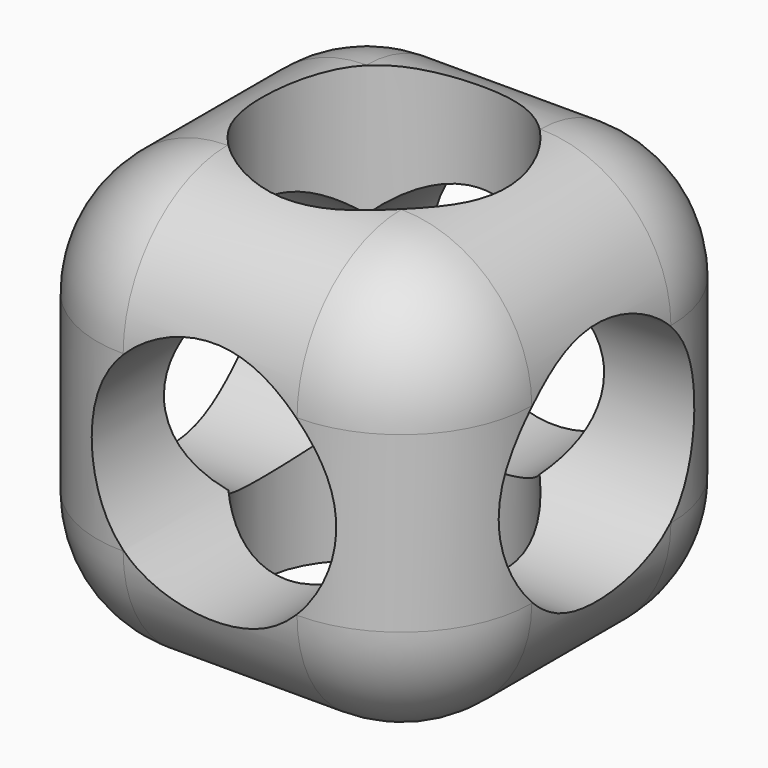
from build123d import *

# Parameters (mm, degrees)
F0_W         = 25.4
F0_H         = 25.4
F1_DEPTH     = 12.7
F5_D         = 14.2875
F5_ON_F3_D   = 14.2875
F5_ON_F2_D   = 14.2875
F6_T1_DEPTH  = 10.16
F6_T3_DEPTH  = 10.16
F6_T5_DEPTH  = 10.16
F6_S9_W      = 7.62
F6_S9_H      = 7.62
F6_T10_DEPTH = 7.62
F6_S15_W     = 7.62
F6_S15_H     = 7.62
F6_T16_DEPTH = 7.62
F6_S21_W     = 7.62
F6_S21_H     = 7.62
F6_T22_DEPTH = 7.62
F6_S27_W     = 7.62
F6_S27_H     = 7.62
F6_T28_DEPTH = 7.62
F6_S33_W     = 7.62
F6_S33_H     = 7.62
F6_T34_DEPTH = 7.62
F6_S39_W     = 7.62
F6_S39_H     = 7.62
F6_T40_DEPTH = 7.62
F6_S45_W     = 7.62
F6_S45_H     = 7.62
F6_T46_DEPTH = 7.62
F6_S51_W     = 7.62
F6_S51_H     = 7.62
F6_T52_DEPTH = 7.62


# Not quite as in the source:
# - a fillet or chamfer that OpenCascade refuses, or shapes differently, is made with other operations: its cross-section is extruded or revolved along the edge and cut away or added
# - a length typed as a fraction of an inch, garbled in the dataset ("3 / 203.2 mm" for 3/8 in), is restored


with BuildPart() as f1:
    # F0 (on Front) → F1 (new body, symmetric)
    with BuildSketch(Plane.XZ):
        Rectangle(F0_W, F0_H)
    extrude(amount=F1_DEPTH, both=True)

    # F5 (through all)
    with Locations(Plane.XY.offset(12.7)):
        with Locations((0, 0)):
            Hole(F5_D / 2)

    # F5 on F3 (through all)
    with Locations(Plane.XZ.offset(12.7)):
        with Locations((0, 0)):
            Hole(F5_ON_F3_D / 2)

    # F5 on F2 (through all)
    with Locations(Plane.YZ.offset(12.7)):
        with Locations((0, 0)):
            Hole(F5_ON_F2_D / 2)

    # F6: fillet of radius 7.62 on 12 edges, made by hand

    # F6_s2 → F6_t1 (cut)
    with BuildSketch(Plane.XZ.offset(-5.08)):
        with BuildLine():
            ThreePointArc((12.7, 5.08), (10.4681536726, 10.4681536726), (5.08, 12.7))
            Line((5.08, 12.7), (12.7, 12.7))
            Line((12.7, 12.7), (12.7, 5.08))
        make_face()
        with BuildLine():
            ThreePointArc((12.7, -5.08), (10.4681536726, -10.4681536726), (5.08, -12.7))
            Line((5.08, -12.7), (12.7, -12.7))
            Line((12.7, -12.7), (12.7, -5.08))
        make_face()
        with BuildLine():
            ThreePointArc((-5.08, 12.7), (-10.4681536726, 10.4681536726), (-12.7, 5.08))
            Line((-12.7, 5.08), (-12.7, 12.7))
            Line((-12.7, 12.7), (-5.08, 12.7))
        make_face()
        with BuildLine():
            ThreePointArc((-5.08, -12.7), (-10.4681536726, -10.4681536726), (-12.7, -5.08))
            Line((-12.7, -5.08), (-12.7, -12.7))
            Line((-12.7, -12.7), (-5.08, -12.7))
        make_face()
    extrude(amount=F6_T1_DEPTH, mode=Mode.SUBTRACT)

    # F6_s4 → F6_t3 (cut)
    with BuildSketch(Plane.XY.offset(-5.08)):
        with BuildLine():
            ThreePointArc((12.7, 5.08), (10.4681536726, 10.4681536726), (5.08, 12.7))
            Line((5.08, 12.7), (12.7, 12.7))
            Line((12.7, 12.7), (12.7, 5.08))
        make_face()
        with BuildLine():
            ThreePointArc((12.7, -5.08), (10.4681536726, -10.4681536726), (5.08, -12.7))
            Line((5.08, -12.7), (12.7, -12.7))
            Line((12.7, -12.7), (12.7, -5.08))
        make_face()
        with BuildLine():
            ThreePointArc((-5.08, -12.7), (-10.4681536726, -10.4681536726), (-12.7, -5.08))
            Line((-12.7, -5.08), (-12.7, -12.7))
            Line((-12.7, -12.7), (-5.08, -12.7))
        make_face()
        with BuildLine():
            ThreePointArc((-5.08, 12.7), (-10.4681536726, 10.4681536726), (-12.7, 5.08))
            Line((-12.7, 5.08), (-12.7, 12.7))
            Line((-12.7, 12.7), (-5.08, 12.7))
        make_face()
    extrude(amount=F6_T3_DEPTH, mode=Mode.SUBTRACT)

    # F6_s6 → F6_t5 (cut)
    with BuildSketch(Plane.YZ.offset(-5.08)):
        with BuildLine():
            ThreePointArc((-5.08, 12.7), (-10.4681536726, 10.4681536726), (-12.7, 5.08))
            Line((-12.7, 5.08), (-12.7, 12.7))
            Line((-12.7, 12.7), (-5.08, 12.7))
        make_face()
        with BuildLine():
            ThreePointArc((-5.08, -12.7), (-10.4681536726, -10.4681536726), (-12.7, -5.08))
            Line((-12.7, -5.08), (-12.7, -12.7))
            Line((-12.7, -12.7), (-5.08, -12.7))
        make_face()
        with BuildLine():
            ThreePointArc((12.7, 5.08), (10.4681536726, 10.4681536726), (5.08, 12.7))
            Line((5.08, 12.7), (12.7, 12.7))
            Line((12.7, 12.7), (12.7, 5.08))
        make_face()
        with BuildLine():
            ThreePointArc((12.7, -5.08), (10.4681536726, -10.4681536726), (5.08, -12.7))
            Line((5.08, -12.7), (12.7, -12.7))
            Line((12.7, -12.7), (12.7, -5.08))
        make_face()
    extrude(amount=F6_T5_DEPTH, mode=Mode.SUBTRACT)


with BuildPart() as f6_tool8:
    # F6_s9 → F6_t10 (new body)
    with BuildSketch(Plane.YZ.offset(5.08)):
        with Locations((8.89, 8.89)):
            Rectangle(F6_S9_W, F6_S9_H)
    extrude(amount=F6_T10_DEPTH)

    # F6_s11 → F6_t12 (revolve, cut)
    with BuildSketch(Plane(origin=(5.08, 5.08, 5.08), x_dir=(0, -0.7071067812, -0.7071067812), z_dir=(0, -0.7071067812, 0.7071067812))):
        with BuildLine():
            ThreePointArc((0, -7.62), (7.62, 0), (0, 7.62))
            Line((0, 7.62), (0, -7.62))
        make_face()
    revolve(axis=Axis((5.08, 5.08, 5.08), (1, 0, 0)), mode=Mode.SUBTRACT)


with BuildPart() as f1_1:
    add(f1.part)

    # F6_t7: cut F6_tool8
    add(f6_tool8.part, mode=Mode.SUBTRACT)


with BuildPart() as f6_tool14:
    # F6_s15 → F6_t16 (new body)
    with BuildSketch(Plane.YZ.offset(5.08)):
        with Locations((-8.89, 8.89)):
            Rectangle(F6_S15_W, F6_S15_H)
    extrude(amount=F6_T16_DEPTH)

    # F6_s17 → F6_t18 (revolve, cut)
    with BuildSketch(Plane(origin=(5.08, -5.08, 5.08), x_dir=(0, 0.7071067812, -0.7071067812), z_dir=(0, -0.7071067812, -0.7071067812))):
        with BuildLine():
            ThreePointArc((0, -7.62), (7.62, 0), (0, 7.62))
            Line((0, 7.62), (0, -7.62))
        make_face()
    revolve(axis=Axis((5.08, -5.08, 5.08), (1, 0, 0)), mode=Mode.SUBTRACT)


with BuildPart() as f1_2:
    add(f1_1.part)

    # F6_t13: cut F6_tool14
    add(f6_tool14.part, mode=Mode.SUBTRACT)


with BuildPart() as f6_tool20:
    # F6_s21 → F6_t22 (new body)
    with BuildSketch(Plane.YZ.offset(5.08)):
        with Locations((-8.89, -8.89)):
            Rectangle(F6_S21_W, F6_S21_H)
    extrude(amount=F6_T22_DEPTH)

    # F6_s23 → F6_t24 (revolve, cut)
    with BuildSketch(Plane(origin=(5.08, -5.08, -5.08), x_dir=(0, 0.7071067812, 0.7071067812), z_dir=(0, 0.7071067812, -0.7071067812))):
        with BuildLine():
            ThreePointArc((0, -7.62), (7.62, 0), (0, 7.62))
            Line((0, 7.62), (0, -7.62))
        make_face()
    revolve(axis=Axis((5.08, -5.08, -5.08), (1, 0, 0)), mode=Mode.SUBTRACT)


with BuildPart() as f1_3:
    add(f1_2.part)

    # F6_t19: cut F6_tool20
    add(f6_tool20.part, mode=Mode.SUBTRACT)


with BuildPart() as f6_tool26:
    # F6_s27 → F6_t28 (new body)
    with BuildSketch(Plane.YZ.offset(5.08)):
        with Locations((8.89, -8.89)):
            Rectangle(F6_S27_W, F6_S27_H)
    extrude(amount=F6_T28_DEPTH)

    # F6_s29 → F6_t30 (revolve, cut)
    with BuildSketch(Plane(origin=(5.08, 5.08, -5.08), x_dir=(0, -0.7071067812, 0.7071067812), z_dir=(0, 0.7071067812, 0.7071067812))):
        with BuildLine():
            ThreePointArc((0, -7.62), (7.62, 0), (0, 7.62))
            Line((0, 7.62), (0, -7.62))
        make_face()
    revolve(axis=Axis((5.08, 5.08, -5.08), (1, 0, 0)), mode=Mode.SUBTRACT)


with BuildPart() as f1_4:
    add(f1_3.part)

    # F6_t25: cut F6_tool26
    add(f6_tool26.part, mode=Mode.SUBTRACT)


with BuildPart() as f6_tool32:
    # F6_s33 → F6_t34 (new body)
    with BuildSketch(Plane.XY.offset(5.08)):
        with Locations((-8.89, -8.89)):
            Rectangle(F6_S33_W, F6_S33_H)
    extrude(amount=F6_T34_DEPTH)

    # F6_s35 → F6_t36 (revolve, cut)
    with BuildSketch(Plane(origin=(-5.08, -5.08, 5.08), x_dir=(0.7071067812, 0.7071067812, 0), z_dir=(0.7071067812, -0.7071067812, 0))):
        with BuildLine():
            ThreePointArc((0, -7.62), (7.62, 0), (0, 7.62))
            Line((0, 7.62), (0, -7.62))
        make_face()
    revolve(axis=Axis((-5.08, -5.08, 5.08), (0, 0, 1)), mode=Mode.SUBTRACT)


with BuildPart() as f1_5:
    add(f1_4.part)

    # F6_t31: cut F6_tool32
    add(f6_tool32.part, mode=Mode.SUBTRACT)


with BuildPart() as f6_tool38:
    # F6_s39 → F6_t40 (new body)
    with BuildSketch(Plane.XY.offset(-5.08)):
        with Locations((-8.89, -8.89)):
            Rectangle(F6_S39_W, F6_S39_H)
    extrude(amount=-F6_T40_DEPTH)

    # F6_s41 → F6_t42 (revolve, cut)
    with BuildSketch(Plane(origin=(-5.08, -5.08, -5.08), x_dir=(0.7071067812, 0.7071067812, 0), z_dir=(-0.7071067812, 0.7071067812, 0))):
        with BuildLine():
            ThreePointArc((0, -7.62), (7.62, 0), (0, 7.62))
            Line((0, 7.62), (0, -7.62))
        make_face()
    revolve(axis=Axis((-5.08, -5.08, -5.08), (0, 0, -1)), mode=Mode.SUBTRACT)


with BuildPart() as f1_6:
    add(f1_5.part)

    # F6_t37: cut F6_tool38
    add(f6_tool38.part, mode=Mode.SUBTRACT)


with BuildPart() as f6_tool44:
    # F6_s45 → F6_t46 (new body)
    with BuildSketch(Plane.XZ.offset(-5.08)):
        with Locations((-8.89, 8.89)):
            Rectangle(F6_S45_W, F6_S45_H)
    extrude(amount=-F6_T46_DEPTH)

    # F6_s47 → F6_t48 (revolve, cut)
    with BuildSketch(Plane(origin=(-5.08, 5.08, 5.08), x_dir=(0.7071067812, 0, -0.7071067812), z_dir=(0.7071067812, 0, 0.7071067812))):
        with BuildLine():
            ThreePointArc((0, -7.62), (7.62, 0), (0, 7.62))
            Line((0, 7.62), (0, -7.62))
        make_face()
    revolve(axis=Axis((-5.08, 5.08, 5.08), (0, 1, 0)), mode=Mode.SUBTRACT)


with BuildPart() as f1_7:
    add(f1_6.part)

    # F6_t43: cut F6_tool44
    add(f6_tool44.part, mode=Mode.SUBTRACT)


with BuildPart() as f6_tool50:
    # F6_s51 → F6_t52 (new body)
    with BuildSketch(Plane.XZ.offset(-5.08)):
        with Locations((-8.89, -8.89)):
            Rectangle(F6_S51_W, F6_S51_H)
    extrude(amount=-F6_T52_DEPTH)

    # F6_s53 → F6_t54 (revolve, cut)
    with BuildSketch(Plane(origin=(-5.08, 5.08, -5.08), x_dir=(0.7071067812, 0, 0.7071067812), z_dir=(-0.7071067812, 0, 0.7071067812))):
        with BuildLine():
            ThreePointArc((0, -7.62), (7.62, 0), (0, 7.62))
            Line((0, 7.62), (0, -7.62))
        make_face()
    revolve(axis=Axis((-5.08, 5.08, -5.08), (0, 1, 0)), mode=Mode.SUBTRACT)


with BuildPart() as f1_8:
    add(f1_7.part)

    # F6_t49: cut F6_tool50
    add(f6_tool50.part, mode=Mode.SUBTRACT)


solid = f1_8.part
